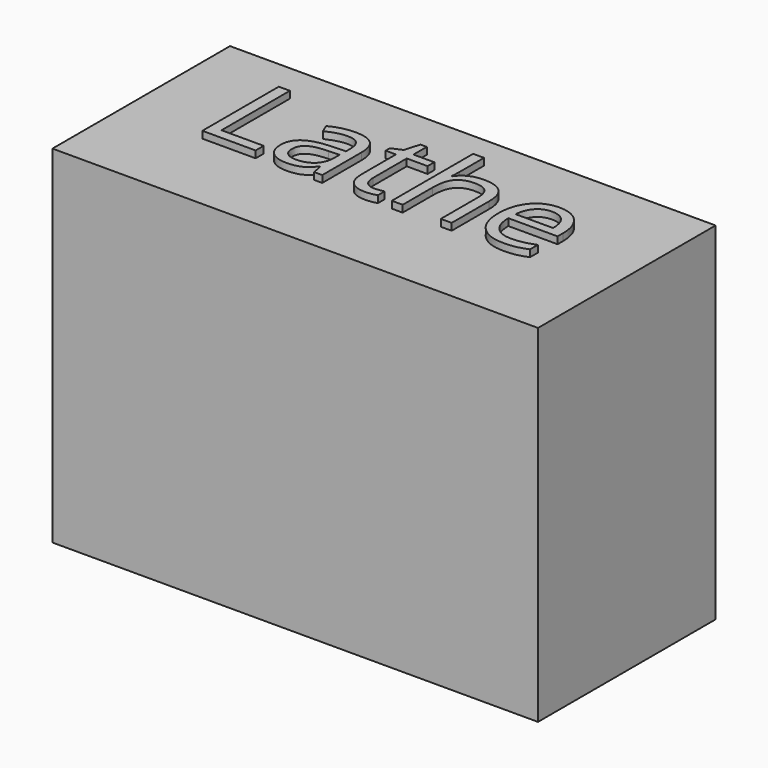
from build123d import *

# Parameters (mm, degrees)
F0_W         = 1778
F0_H         = 812.8
F1_DEPTH     = 1270
F2_TEXT_SIZE = 489.9406598674
F3_DEPTH     = 25.4


# Not quite as in the source:
# - Text() gives the source's letters only with a copy of the font that has no kerning and outlines rounded to 1/6400 em; it was checked with that copy


with BuildPart() as f1:
    # F0 (on Top) → F1 (new body)
    with BuildSketch(Plane.XY):
        Rectangle(F0_W, F0_H)
    extrude(amount=F1_DEPTH)

    # F2 (on face) → F3 (join)
    with BuildSketch(Plane.XY.offset(1270)):
        with Locations((-640.7122426188, -90.6314849854)):
            Text('Lathe', F2_TEXT_SIZE, font='Open Sans', text_align=(TextAlign.LEFT, TextAlign.BOTTOM))
    extrude(amount=F3_DEPTH)


solid = f1.part
